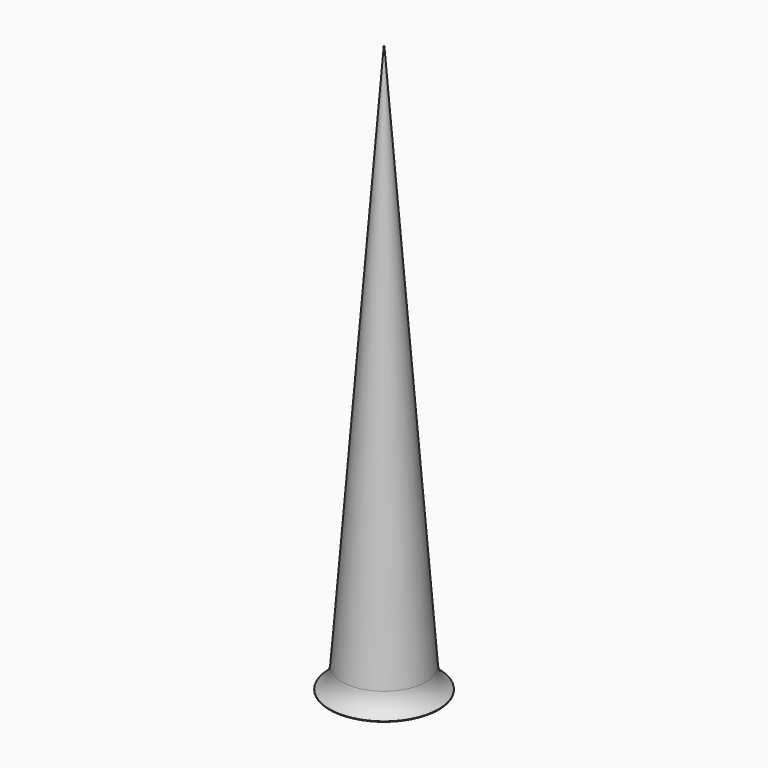
from build123d import *

# Parameters (mm, degrees)
F0_R     = 85
F2_R     = 0.5
F4_R     = 105.9677495378
F5_DEPTH = 1


# Not quite as in the source:
# - a fillet or chamfer that OpenCascade refuses, or shapes differently, is made with other operations: its cross-section is extruded or revolved along the edge and cut away or added


with BuildPart() as f3:
    # F0 (on Top) → F3 section 0
    with BuildSketch(Plane.XY):
        Circle(F0_R)
    # F2 (on offset) → F3 section 1
    with BuildSketch(Plane.XY.offset(1100)):
        Circle(F2_R)
    loft()

    # F4 (on Top) → F5 (join)
    with BuildSketch(Plane.XY):
        Circle(F4_R)
    extrude(amount=F5_DEPTH)

    # F6: fillet of radius 50 on 1 edges, made by hand


with BuildPart() as f6_tool2:
    # F6_s3 → F6_t4 (revolve)
    with BuildSketch(Plane.XZ):
        with BuildLine():
            ThreePointArc((105.9675430277, 0.9996574309), (89.2196248611, 17.5811287524), (81.9274601503, 39.9923377321))
            Line((81.9274601503, 39.9923377321), (76.9419980029, 39.6093635944))
            ThreePointArc((76.9419980029, 39.6093635944), (78.4400582493, 20.1132100469), (79.9377196708, 0.6170258623))
            Line((79.9377196708, 0.6170258623), (84.9231818182, -4.0001501991))
            ThreePointArc((84.9231818182, -4.0001501991), (95.4453624229, -4.0001501991), (103.386089168, -3.2825847369))
            Line((103.386089168, -3.2825847369), (105.9675430277, 0.9996574309))
        make_face()
    revolve(axis=Axis((0, 0, 1), (0, 0, 1)))

    split(bisect_by=Plane.XY, keep=Keep.TOP)


with BuildPart() as f3_1:
    add(f3.part)

    # F6_t1: union F6_tool2
    add(f6_tool2.part)


solid = f3_1.part
